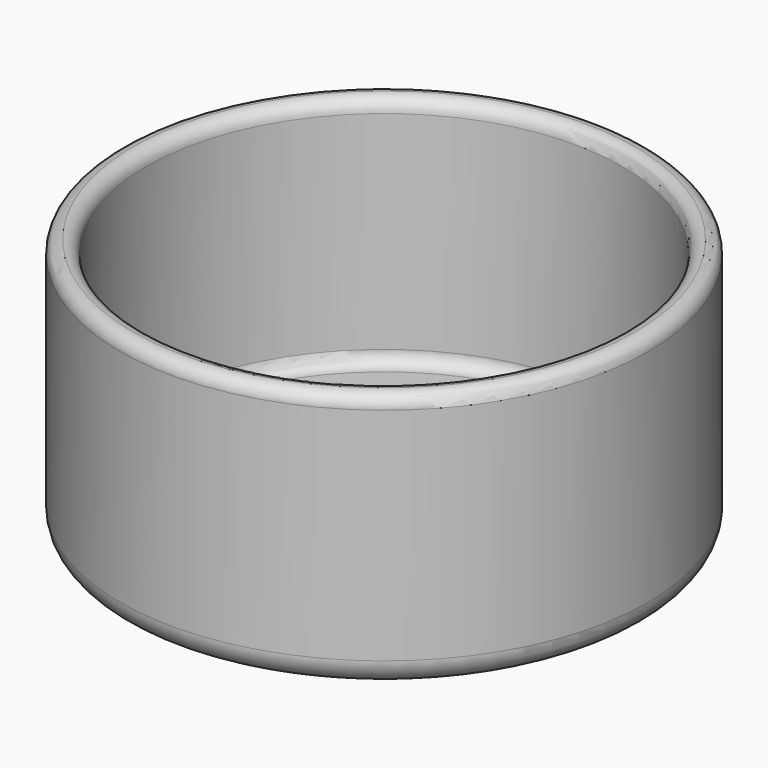
from build123d import *

# Parameters (mm, degrees)
F0_R     = 30.5
F0_R_2   = 27.5
F1_DEPTH = 27
F2_DEPTH = 3
F3_R     = 1.49999
F4_R     = 2.99999


# Not quite as in the source:
# - a fillet or chamfer is up to 0.001 mm smaller than in the source, because OpenCascade refuses the exact size


with BuildPart() as f1:
    # F0 (on Top) → F1 (new body)
    with BuildSketch(Plane.XY):
        Circle(F0_R)
        Circle(F0_R_2, mode=Mode.SUBTRACT)
    extrude(amount=F1_DEPTH)

    # F0 (on Top) → F2 (join)
    with BuildSketch(Plane.XY):
        Circle(F0_R)
        Circle(F0_R_2, mode=Mode.SUBTRACT)
        Circle(F0_R_2)
    extrude(amount=-F2_DEPTH)

    # F3 (radius 1.5 in the source; OpenCascade refuses exactly that, so slightly less here)
    f3_edges = [f1.edges().sort_by_distance(p)[0] for p in [
        (-30.5, 0, 27),
        (-27.5, 0, 27),
        (-27.5, 0, 0),
    ]]
    fillet(f3_edges, radius=F3_R)

    # F4 (radius 3 in the source; OpenCascade refuses exactly that, so slightly less here)
    f4_edges = [f1.edges().sort_by_distance(p)[0] for p in [
        (-30.5, 0, -3),
    ]]
    fillet(f4_edges, radius=F4_R)


solid = f1.part
